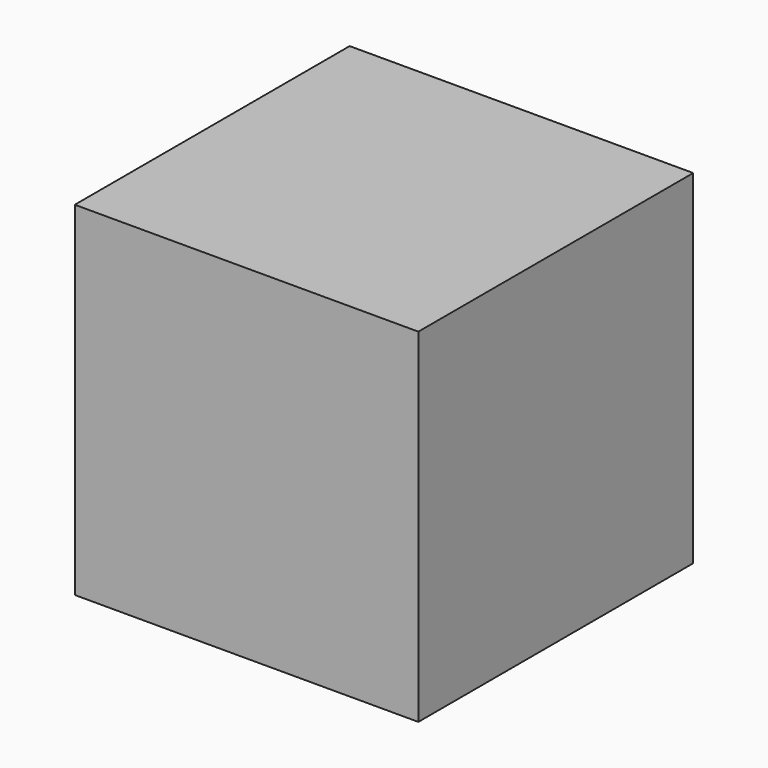
from build123d import *

# Parameters (mm, degrees)
F0_W     = 76.2
F0_H     = 76.2
F2_DEPTH = 76.2


# Not quite as in the source:
# - the program builds the solid bodies; features that only make, move or delete a surface that nothing else refers to are left out


with BuildPart() as f2:
    # F0 (on Top) → F2 (new body)
    with BuildSketch(Plane.XY):
        Rectangle(F0_W, F0_H)
    extrude(amount=F2_DEPTH)


solid = f2.part
